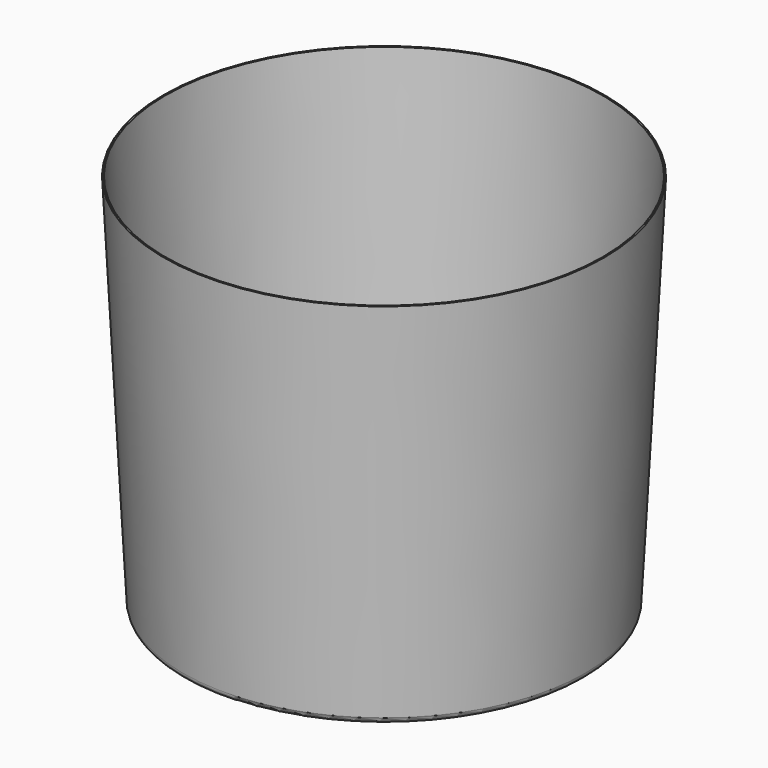
from build123d import *

# Parameters (mm, degrees)
F2_R = 1025
F0_R = 935
F4_R = 30
F5_T = -7


with BuildPart() as f3:
    # F2 (on offset) → F3 section 0
    with BuildSketch(Plane.XY.offset(1760)):
        Circle(F2_R)
    # F0 (on Top) → F3 section 1
    with BuildSketch(Plane.XY):
        Circle(F0_R)
    loft()

    # F4
    f4_edges = [f3.edges().sort_by_distance(p)[0] for p in [
        (-935, 0, 0),
    ]]
    fillet(f4_edges, radius=F4_R)

    # F5
    f5_openings = [f3.faces().sort_by_distance(p)[0] for p in [
        (0, 0, 1760),
    ]]
    offset(amount=F5_T, openings=f5_openings, kind=Kind.INTERSECTION)


solid = f3.part
